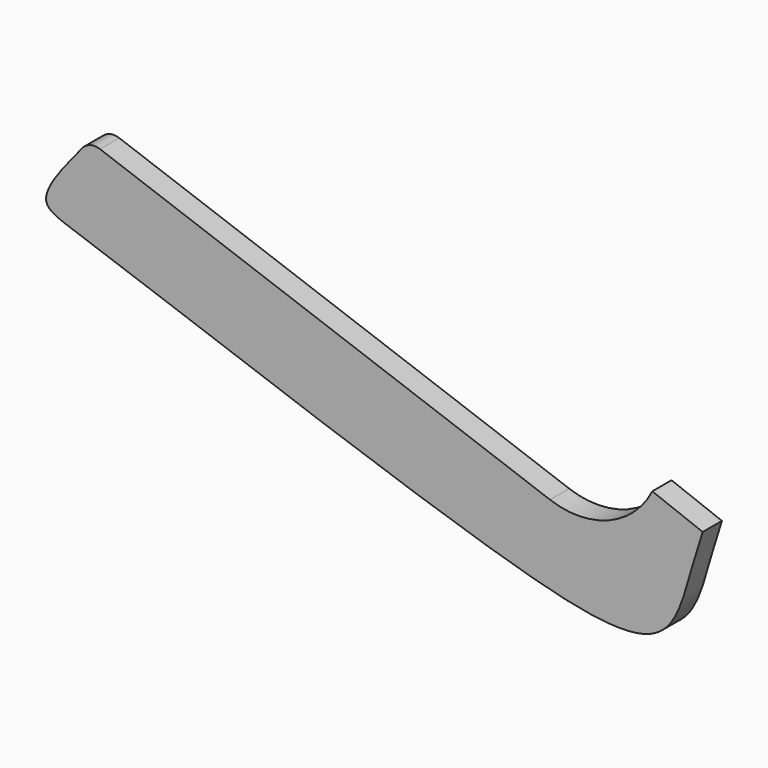
from build123d import *

# Parameters (mm, degrees)
F1_DEPTH = 19.05


with BuildPart() as f1:
    # F0 (on Front) → F1 (new body)
    with BuildSketch(Plane.XZ):
        with BuildLine():
            Line((51.3480285322, -86.7852984616), (-305.3616061666, 41.9014199259))
            ThreePointArc((-305.3616061666, 41.9014199259), (-312.981533952, 42.2160798285), (-319.4077985163, 38.1093251416))
            add(Edge.make_bspline(
                [(172.4495707126, -69.9309047478), (170.7565397374, -74.8879578834), (159.6172151028, -109.2209226086), (149.008066375, -172.0943551046), (5.705430346, -143.7182399989), (-308.8758408469, -25.714201087), (-359.3207511694, -11.2848664797), (-334.5650047362, 20.0112367074), (-319.4077985163, 38.1093251416)],
                knots=[0.7762192949, 0.7762192949, 0.7762192949, 0.7762192949, 0.7821011157, 0.8175501575, 0.8647494322, 0.9431559258, 0.9670432321, 0.9963460987, 0.9963460987, 0.9963460987, 0.9963460987], degree=3))
            Line((172.4495707126, -69.9309047478), (132.4956117337, -54.5537738749))
            ThreePointArc((132.4956117337, -54.5537738749), (98.0275737575, -86.0416650579), (51.3480285322, -86.7852984616))
        make_face()
    extrude(amount=F1_DEPTH)


solid = f1.part
